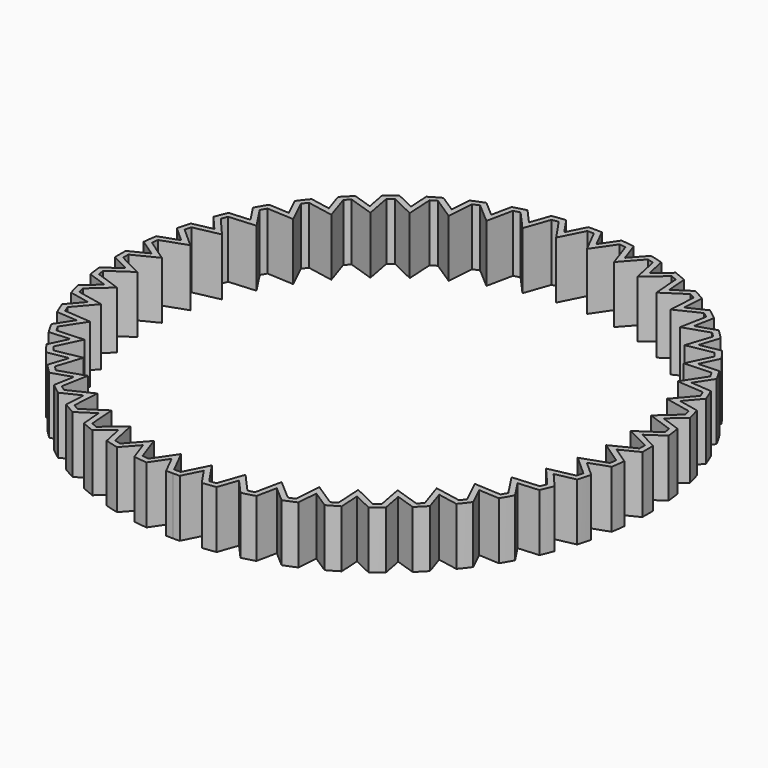
from build123d import *

# Parameters (mm, degrees)
F2_DEPTH = 5.1


# Not quite as in the source:
# - ends of sketch curves that miss each other by under 0.0002 mm in the source are joined


with BuildPart() as f2:
    # F1 (on Top) → F2 (new body, symmetric)
    with BuildSketch(Plane.XY):
        with BuildLine():
            Line((-46.740944, 4.935179), (-43.707361, 2.864732))
            Line((-43.707361, 2.864732), (-46.985243, 1.207778))
            Line((-46.985243, 1.207778), (-46.985243, 0))
            Line((-46.985243, 0), (-46.985243, -1.207778))
            Line((-46.985243, -1.207778), (-43.707361, -2.864732))
            Line((-43.707361, -2.864732), (-46.740944, -4.935179))
            ThreePointArc((-46.740944, -4.935179), (-46.5986899783, -6.134650804), (-46.4256600093, -7.3300710015))
            Line((-46.4256600093, -7.3300710015), (-42.959516, -8.545179))
            Line((-42.959516, -8.545179), (-45.696856, -10.994052))
            ThreePointArc((-45.696856, -10.994052), (-45.3992520814, -12.1646931171), (-45.0716642771, -13.3273000819))
            Line((-45.0716642771, -13.3273000819), (-41.476621, -14.079416))
            Line((-41.476621, -14.079416), (-43.870901, -16.864633))
            ThreePointArc((-43.870901, -16.864633), (-43.4230440531, -17.9864141326), (-42.9465081363, -19.0963160606))
            Line((-42.9465081363, -19.0963160606), (-39.284051, -19.37275))
            Line((-39.284051, -19.37275), (-41.294303, -22.446655))
            ThreePointArc((-41.294303, -22.446655), (-40.7038559026, -23.5003821851), (-40.0865255496, -24.5385883364))
            Line((-40.0865255496, -24.5385883364), (-36.419319, -24.334611))
            Line((-36.419319, -24.334611), (-38.011148, -27.644609))
            ThreePointArc((-38.011148, -27.644609), (-37.2882132363, -28.6122526522), (-36.5406510894, -29.5609990723))
            Line((-36.5406510894, -29.5609990723), (-32.931442, -28.8801))
            Line((-32.931442, -28.8801), (-34.077612, -32.369556))
            ThreePointArc((-34.077612, -32.369556), (-33.2345591831, -33.2345591831), (-32.3695563878, -34.0776124082))
            Line((-32.3695563878, -34.0776124082), (-28.8801, -32.931442))
            Line((-28.8801, -32.931442), (-29.5609988987, -36.540650463))
            ThreePointArc((-29.5609988987, -36.540650463), (-28.6122526522, -37.2882132363), (-27.6446094326, -38.0111485949))
            Line((-27.6446094326, -38.0111485949), (-24.334611, -36.419319))
            Line((-24.334611, -36.419319), (-24.5385880151, -40.086525271))
            ThreePointArc((-24.5385880151, -40.086525271), (-23.5003821851, -40.7038559026), (-22.4466553416, -41.2943036285))
            Line((-22.4466553416, -41.2943036285), (-19.37275, -39.284051))
            Line((-19.37275, -39.284051), (-19.0963160124, -42.9465078358))
            ThreePointArc((-19.0963160124, -42.9465078358), (-17.9864141326, -43.4230440531), (-16.864633181, -43.8709014708))
            Line((-16.864633181, -43.8709014708), (-14.079416, -41.476621))
            Line((-14.079416, -41.476621), (-13.3272999873, -45.0716640609))
            ThreePointArc((-13.3272999873, -45.0716640609), (-12.1646931171, -45.3992520814), (-10.9940520511, -45.6968562123))
            Line((-10.9940520511, -45.6968562123), (-8.545179, -42.959516))
            Line((-8.545179, -42.959516), (-7.3302500727, -46.4256317925))
            ThreePointArc((-7.3302500727, -46.4256317925), (-6.1348308361, -46.598666277), (-4.93536, -46.740925))
            Line((-4.93536, -46.740925), (-2.864732, -43.707361))
            Line((-2.864732, -43.707361), (-1.2077776691, -46.9852436547))
            Line((-1.2077776691, -46.9852436547), (0, -47.0162901536))
            Line((0, -47.0162901536), (1.2077776691, -46.9852436547))
            Line((1.2077776691, -46.9852436547), (2.864732, -43.707361))
            Line((2.864732, -43.707361), (4.93536, -46.740925))
            ThreePointArc((4.93536, -46.740925), (6.1348308361, -46.598666277), (7.330249961, -46.4256317533))
            Line((7.330249961, -46.4256317533), (8.545179, -42.959516))
            Line((8.545179, -42.959516), (10.994052, -45.696856))
            ThreePointArc((10.994052, -45.696856), (12.1646931171, -45.3992520814), (13.3273000819, -45.0716642771))
            Line((13.3273000819, -45.0716642771), (14.079416, -41.476621))
            Line((14.079416, -41.476621), (16.8646331123, -43.8709010965))
            ThreePointArc((16.8646331123, -43.8709010965), (17.9864141326, -43.4230440531), (19.0963160606, -42.9465081363))
            Line((19.0963160606, -42.9465081363), (19.37275, -39.284051))
            Line((19.37275, -39.284051), (22.4466552794, -41.2943031827))
            ThreePointArc((22.4466552794, -41.2943031827), (23.5003821851, -40.7038559026), (24.5385883364, -40.0865255496))
            Line((24.5385883364, -40.0865255496), (24.334611, -36.419319))
            Line((24.334611, -36.419319), (27.644609, -38.011148))
            ThreePointArc((27.644609, -38.011148), (28.6122526522, -37.2882132363), (29.5609990723, -36.5406510894))
            Line((29.5609990723, -36.5406510894), (28.8801, -32.931442))
            Line((28.8801, -32.931442), (32.369556, -34.077612))
            ThreePointArc((32.369556, -34.077612), (33.2345591831, -33.2345591831), (34.0776124082, -32.3695563878))
            Line((34.0776124082, -32.3695563878), (32.931442, -28.8801))
            Line((32.931442, -28.8801), (36.540651, -29.560999))
            ThreePointArc((36.540651, -29.560999), (37.2882132363, -28.6122526522), (38.0111485949, -27.6446094326))
            Line((38.0111485949, -27.6446094326), (36.419319, -24.334611))
            Line((36.419319, -24.334611), (40.086525, -24.538588))
            ThreePointArc((40.086525, -24.538588), (40.7038559026, -23.5003821851), (41.2943036285, -22.4466553416))
            Line((41.2943036285, -22.4466553416), (39.284051, -19.37275))
            Line((39.284051, -19.37275), (42.946508, -19.096316))
            ThreePointArc((42.946508, -19.096316), (43.4230440531, -17.9864141326), (43.8709014708, -16.864633181))
            Line((43.8709014708, -16.864633181), (41.476621, -14.079416))
            Line((41.476621, -14.079416), (45.071664, -13.3273))
            ThreePointArc((45.071664, -13.3273), (45.3992520814, -12.1646931171), (45.6968562123, -10.9940520511))
            Line((45.6968562123, -10.9940520511), (42.959516, -8.545179))
            Line((42.959516, -8.545179), (46.42566, -7.330071))
            ThreePointArc((46.42566, -7.330071), (46.5986899783, -6.134650804), (46.7409441102, -4.9351790116))
            Line((46.7409441102, -4.9351790116), (43.707361, -2.864732))
            Line((43.707361, -2.864732), (46.985243, -1.207778))
            Line((46.985243, -1.207778), (46.985243, 0))
            Line((46.985243, 0), (46.985243, 1.207778))
            Line((46.985243, 1.207778), (43.707361, 2.864732))
            Line((43.707361, 2.864732), (46.740944, 4.935179))
            ThreePointArc((46.740944, 4.935179), (46.5986899783, 6.134650804), (46.4256600093, 7.3300710015))
            Line((46.4256600093, 7.3300710015), (42.959516, 8.545179))
            Line((42.959516, 8.545179), (45.696856, 10.994052))
            ThreePointArc((45.696856, 10.994052), (45.3992520814, 12.1646931171), (45.0716642771, 13.3273000819))
            Line((45.0716642771, 13.3273000819), (41.476621, 14.079416))
            Line((41.476621, 14.079416), (43.870901, 16.864633))
            ThreePointArc((43.870901, 16.864633), (43.4230440531, 17.9864141326), (42.9465081363, 19.0963160606))
            Line((42.9465081363, 19.0963160606), (39.284051, 19.37275))
            Line((39.284051, 19.37275), (41.294303, 22.446655))
            ThreePointArc((41.294303, 22.446655), (40.7038559026, 23.5003821851), (40.0865255496, 24.5385883364))
            Line((40.0865255496, 24.5385883364), (36.419319, 24.334611))
            Line((36.419319, 24.334611), (38.011148, 27.644609))
            ThreePointArc((38.011148, 27.644609), (37.2882132363, 28.6122526522), (36.5406510894, 29.5609990723))
            Line((36.5406510894, 29.5609990723), (32.931442, 28.8801))
            Line((32.931442, 28.8801), (34.077612, 32.369556))
            ThreePointArc((34.077612, 32.369556), (33.2345591831, 33.2345591831), (32.3695563878, 34.0776124082))
            Line((32.3695563878, 34.0776124082), (28.8801, 32.931442))
            Line((28.8801, 32.931442), (29.5609988987, 36.540650463))
            ThreePointArc((29.5609988987, 36.540650463), (28.6122526522, 37.2882132363), (27.6446094326, 38.0111485949))
            Line((27.6446094326, 38.0111485949), (24.334611, 36.419319))
            Line((24.334611, 36.419319), (24.5385880151, 40.086525271))
            ThreePointArc((24.5385880151, 40.086525271), (23.5003821851, 40.7038559026), (22.4466553416, 41.2943036285))
            Line((22.4466553416, 41.2943036285), (19.37275, 39.284051))
            Line((19.37275, 39.284051), (19.0963160124, 42.9465078358))
            ThreePointArc((19.0963160124, 42.9465078358), (17.9864141326, 43.4230440531), (16.864633181, 43.8709014708))
            Line((16.864633181, 43.8709014708), (14.079416, 41.476621))
            Line((14.079416, 41.476621), (13.3272999873, 45.0716640609))
            ThreePointArc((13.3272999873, 45.0716640609), (12.1646931171, 45.3992520814), (10.9940520511, 45.6968562123))
            Line((10.9940520511, 45.6968562123), (8.545179, 42.959516))
            Line((8.545179, 42.959516), (7.3302500727, 46.4256317925))
            ThreePointArc((7.3302500727, 46.4256317925), (6.1348308361, 46.598666277), (4.93536, 46.740925))
            Line((4.93536, 46.740925), (2.864732, 43.707361))
            Line((2.864732, 43.707361), (1.2077776691, 46.9852436547))
            Line((1.2077776691, 46.9852436547), (0, 47.0162901536))
            Line((0, 47.0162901536), (-1.2077776691, 46.9852436547))
            Line((-1.2077776691, 46.9852436547), (-2.8647316691, 43.7073616547))
            Line((-2.8647316691, 43.7073616547), (-4.93536, 46.740925))
            ThreePointArc((-4.93536, 46.740925), (-6.1348308361, 46.598666277), (-7.330249961, 46.4256317533))
            Line((-7.330249961, 46.4256317533), (-8.545179, 42.959516))
            Line((-8.545179, 42.959516), (-10.994052, 45.696856))
            ThreePointArc((-10.994052, 45.696856), (-12.1646930606, 45.3992518705), (-13.32730002, 45.0716640678))
            Line((-13.32730002, 45.0716640678), (-14.079416, 41.476621))
            Line((-14.079416, 41.476621), (-16.864633, 43.870901))
            ThreePointArc((-16.864633, 43.870901), (-17.9864140039, 43.4230437425), (-19.096315924, 42.9465078291))
            Line((-19.096315924, 42.9465078291), (-19.37275, 39.284051))
            Line((-19.37275, 39.284051), (-22.446655, 41.294303))
            ThreePointArc((-22.446655, 41.294303), (-23.500382017, 40.7038556115), (-24.5385881609, 40.0865252629))
            Line((-24.5385881609, 40.0865252629), (-24.334611, 36.419319))
            Line((-24.334611, 36.419319), (-27.644609, 38.011148))
            ThreePointArc((-27.644609, 38.011148), (-28.6122522044, 37.2882126527), (-29.5609986097, 36.5406505175))
            Line((-29.5609986097, 36.5406505175), (-28.8801, 32.931442))
            Line((-28.8801, 32.931442), (-32.369556, 34.077612))
            ThreePointArc((-32.369556, 34.077612), (-33.2345589453, 33.2345589453), (-34.0776121645, 32.3695561562))
            Line((-34.0776121645, 32.3695561562), (-32.931442, 28.8801))
            Line((-32.931442, 28.8801), (-36.540651, 29.560999))
            ThreePointArc((-36.540651, 29.560999), (-37.2882131451, 28.6122525822), (-38.0111485019, 27.644609365))
            Line((-38.0111485019, 27.644609365), (-36.419319, 24.334611))
            Line((-36.419319, 24.334611), (-40.086525, 24.538588))
            ThreePointArc((-40.086525, 24.538588), (-40.7038556115, 23.500382017), (-41.2943033331, 22.4466551811))
            Line((-41.2943033331, 22.4466551811), (-39.284051, 19.37275))
            Line((-39.284051, 19.37275), (-42.946508, 19.096316))
            ThreePointArc((-42.946508, 19.096316), (-43.4230439153, 17.9864140755), (-43.8709013315, 16.8646331275))
            Line((-43.8709013315, 16.8646331275), (-41.476621, 14.079416))
            Line((-41.476621, 14.079416), (-45.071664, 13.3273))
            ThreePointArc((-45.071664, 13.3273), (-45.3992517567, 12.1646930301), (-45.6968558854, 10.9940519724))
            Line((-45.6968558854, 10.9940519724), (-42.959516, 8.545179))
            Line((-42.959516, 8.545179), (-46.42566, 7.330071))
            ThreePointArc((-46.42566, 7.330071), (-46.598689645, 6.1346507601), (-46.740944, 4.935179))
        make_face()
        with BuildLine():
            Line((-5.4220195115, 45.6801049272), (-2.7361214918, 41.7451424229))
            Line((-2.7361214918, 41.7451424229), (-0.5869250263, 45.9968068679))
            Line((-0.5869250263, 45.9968068679), (0, 45.9968068679))
            Line((0, 45.9968068679), (0.5869250263, 45.9968068679))
            Line((0.5869250263, 45.9968068679), (2.7361214918, 41.7451424229))
            Line((2.7361214918, 41.7451424229), (5.4220195115, 45.6801049272))
            ThreePointArc((5.4220195115, 45.6801049272), (6.0043046559, 45.607221), (6.5856126633, 45.52691498))
            Line((6.5856126633, 45.52691498), (8.1615477089, 41.0308714443))
            Line((8.1615477089, 41.0308714443), (11.3380832459, 44.5815895855))
            ThreePointArc((11.3380832459, 44.5815895855), (11.9058739168, 44.4333258717), (12.4717269771, 44.2778308858))
            Line((12.4717269771, 44.2778308858), (13.4473280598, 39.6145499373))
            Line((13.4473280598, 39.6145499373), (17.0601497389, 42.7202708524))
            ThreePointArc((17.0601497389, 42.7202708524), (17.6037306142, 42.4991641119), (18.1444465413, 42.2711407636))
            Line((18.1444465413, 42.2711407636), (18.5030205002, 37.5204144542))
            Line((18.5030205002, 37.5204144542), (22.4903118144, 40.1279967767))
            ThreePointArc((22.4903118144, 40.1279967767), (23.0003819809, 39.8378301427), (23.506708912, 39.5411800263))
            Line((23.506708912, 39.5411800263), (23.2421216274, 34.7842931877))
            Line((23.2421216274, 34.7842931877), (27.5356584306, 36.849121141))
            ThreePointArc((27.5356584306, 36.849121141), (28.0034910581, 36.4948595052), (28.4667659651, 36.1346581171))
            Line((28.4667659651, 36.1346581171), (27.5835430367, 31.4530021111))
            Line((27.5835430367, 31.4530021111), (32.109862911, 32.9397473374))
            ThreePointArc((32.109862911, 32.9397473374), (32.5274521116, 32.5274521116), (32.9397475781, 32.1098631457))
            Line((32.9397475781, 32.1098631457), (31.4530021111, 27.5835430367))
            Line((31.4530021111, 27.5835430367), (36.1346582271, 28.4667656396))
            ThreePointArc((36.1346582271, 28.4667656396), (36.4948595052, 28.0034910581), (36.8491215365, 27.5356591302))
            Line((36.8491215365, 27.5356591302), (34.7842931877, 23.2421216274))
            Line((34.7842931877, 23.2421216274), (39.5411797373, 23.5067087403))
            ThreePointArc((39.5411797373, 23.5067087403), (39.8378301427, 23.0003819809), (40.1279970699, 22.4903119788))
            Line((40.1279970699, 22.4903119788), (37.5204144542, 18.5030205002))
            Line((37.5204144542, 18.5030205002), (42.271140665, 18.1444463929))
            ThreePointArc((42.271140665, 18.1444463929), (42.4991641119, 17.6037306142), (42.7202711284, 17.0601499542))
            Line((42.7202711284, 17.0601499542), (39.6145499373, 13.4473280598))
            Line((39.6145499373, 13.4473280598), (44.2778305456, 12.4717269452))
            ThreePointArc((44.2778305456, 12.4717269452), (44.4333258717, 11.9058739168), (44.5815898122, 11.3380832401))
            Line((44.5815898122, 11.3380832401), (41.0309340793, 8.1616037433))
            Line((41.0309340793, 8.1616037433), (45.5269361782, 6.585463768))
            ThreePointArc((45.5269361782, 6.585463768), (45.6072406867, 6.0041551186), (45.6801227556, 5.4218693069))
            Line((45.6801227556, 5.4218693069), (41.7450671545, 2.7361595396))
            Line((41.7450671545, 2.7361595396), (45.9969190154, 0.5868683362))
            Line((45.9969190154, 0.5868683362), (45.9969190154, 0))
            Line((45.9969190154, 0), (45.9969190154, -0.5868683362))
            Line((45.9969190154, -0.5868683362), (41.7450671545, -2.7361595396))
            Line((41.7450671545, -2.7361595396), (45.6801224217, -5.4218692673))
            ThreePointArc((45.6801224217, -5.4218692673), (45.6072406867, -6.0041551186), (45.526936511, -6.5854638161))
            Line((45.526936511, -6.5854638161), (41.0309340793, -8.1616037433))
            Line((41.0309340793, -8.1616037433), (44.5815894864, -11.3380831572))
            ThreePointArc((44.5815894864, -11.3380831572), (44.4333258717, -11.9058739168), (44.2778308692, -12.4717270363))
            Line((44.2778308692, -12.4717270363), (39.6145499373, -13.4473280598))
            Line((39.6145499373, -13.4473280598), (42.7202709899, -17.0601498989))
            ThreePointArc((42.7202709899, -17.0601498989), (42.4991641119, -17.6037306142), (42.2711408021, -18.1444464517))
            Line((42.2711408021, -18.1444464517), (37.5204144542, -18.5030205002))
            Line((37.5204144542, -18.5030205002), (40.1279967767, -22.4903118144))
            ThreePointArc((40.1279967767, -22.4903118144), (39.8378301427, -23.0003819809), (39.5411800263, -23.506708912))
            Line((39.5411800263, -23.506708912), (34.7842931877, -23.2421216274))
            Line((34.7842931877, -23.2421216274), (36.8491214444, -27.5356590614))
            ThreePointArc((36.8491214444, -27.5356590614), (36.4948595052, -28.0034910581), (36.1346583174, -28.4667657108))
            Line((36.1346583174, -28.4667657108), (31.4530021111, -27.5835430367))
            Line((31.4530021111, -27.5835430367), (32.9397473374, -32.109862911))
            ThreePointArc((32.9397473374, -32.109862911), (32.5274521116, -32.5274521116), (32.1098631457, -32.9397475781))
            Line((32.1098631457, -32.9397475781), (27.5835430367, -31.4530021111))
            Line((27.5835430367, -31.4530021111), (28.4667655099, -36.1346575392))
            ThreePointArc((28.4667655099, -36.1346575392), (28.0034910581, -36.4948595052), (27.5356588709, -36.8491217303))
            Line((27.5356588709, -36.8491217303), (23.2421216274, -34.7842931877))
            Line((23.2421216274, -34.7842931877), (23.5067087403, -39.5411797373))
            ThreePointArc((23.5067087403, -39.5411797373), (23.0003819809, -39.8378301427), (22.4903119788, -40.1279970699))
            Line((22.4903119788, -40.1279970699), (18.5030205002, -37.5204144542))
            Line((18.5030205002, -37.5204144542), (18.1444464087, -42.2711404547))
            ThreePointArc((18.1444464087, -42.2711404547), (17.6037306142, -42.4991641119), (17.0601498636, -42.7202711646))
            Line((17.0601498636, -42.7202711646), (13.4473280598, -39.6145499373))
            Line((13.4473280598, -39.6145499373), (12.471726918, -44.2778306757))
            ThreePointArc((12.471726918, -44.2778306757), (11.9058739168, -44.4333258717), (11.3380832997, -44.5815897971))
            Line((11.3380832997, -44.5815897971), (8.1615477089, -41.0308714443))
            Line((8.1615477089, -41.0308714443), (6.5856126633, -45.52691498))
            ThreePointArc((6.5856126633, -45.52691498), (6.0043046559, -45.607221), (5.4220195115, -45.6801049272))
            Line((5.4220195115, -45.6801049272), (2.7361214918, -41.7451424229))
            Line((2.7361214918, -41.7451424229), (0.5869250263, -45.9968068679))
            Line((0.5869250263, -45.9968068679), (0, -45.9968068679))
            Line((0, -45.9968068679), (-0.5869250263, -45.9968068679))
            Line((-0.5869250263, -45.9968068679), (-2.7361214918, -41.7451424229))
            Line((-2.7361214918, -41.7451424229), (-5.4220195115, -45.6801049272))
            ThreePointArc((-5.4220195115, -45.6801049272), (-6.0043046559, -45.607221), (-6.5856126633, -45.52691498))
            Line((-6.5856126633, -45.52691498), (-8.1615477089, -41.0308714443))
            Line((-8.1615477089, -41.0308714443), (-11.3380832459, -44.5815895855))
            ThreePointArc((-11.3380832459, -44.5815895855), (-11.9058739168, -44.4333258717), (-12.4717269771, -44.2778308858))
            Line((-12.4717269771, -44.2778308858), (-13.4473280598, -39.6145499373))
            Line((-13.4473280598, -39.6145499373), (-17.0601497389, -42.7202708524))
            ThreePointArc((-17.0601497389, -42.7202708524), (-17.6037306142, -42.4991641119), (-18.1444465413, -42.2711407636))
            Line((-18.1444465413, -42.2711407636), (-18.5030205002, -37.5204144542))
            Line((-18.5030205002, -37.5204144542), (-22.4903118144, -40.1279967767))
            ThreePointArc((-22.4903118144, -40.1279967767), (-23.0003819809, -39.8378301427), (-23.506708912, -39.5411800263))
            Line((-23.506708912, -39.5411800263), (-23.2421216274, -34.7842931877))
            Line((-23.2421216274, -34.7842931877), (-27.5356584306, -36.849121141))
            ThreePointArc((-27.5356584306, -36.849121141), (-28.0034910581, -36.4948595052), (-28.4667659651, -36.1346581171))
            Line((-28.4667659651, -36.1346581171), (-27.5835430367, -31.4530021111))
            Line((-27.5835430367, -31.4530021111), (-32.109862911, -32.9397473374))
            ThreePointArc((-32.109862911, -32.9397473374), (-32.5274521116, -32.5274521116), (-32.9397475781, -32.1098631457))
            Line((-32.9397475781, -32.1098631457), (-31.4530021111, -27.5835430367))
            Line((-31.4530021111, -27.5835430367), (-36.1346582271, -28.4667656396))
            ThreePointArc((-36.1346582271, -28.4667656396), (-36.4948595052, -28.0034910581), (-36.8491215365, -27.5356591302))
            Line((-36.8491215365, -27.5356591302), (-34.7842931877, -23.2421216274))
            Line((-34.7842931877, -23.2421216274), (-39.5411797373, -23.5067087403))
            ThreePointArc((-39.5411797373, -23.5067087403), (-39.8378301427, -23.0003819809), (-40.1279970699, -22.4903119788))
            Line((-40.1279970699, -22.4903119788), (-37.5204144542, -18.5030205002))
            Line((-37.5204144542, -18.5030205002), (-42.271140665, -18.1444463929))
            ThreePointArc((-42.271140665, -18.1444463929), (-42.4991641119, -17.6037306142), (-42.7202711284, -17.0601499542))
            Line((-42.7202711284, -17.0601499542), (-39.6145499373, -13.4473280598))
            Line((-39.6145499373, -13.4473280598), (-44.2778305456, -12.4717269452))
            ThreePointArc((-44.2778305456, -12.4717269452), (-44.4333258717, -11.9058739168), (-44.5815898122, -11.3380832401))
            Line((-44.5815898122, -11.3380832401), (-41.0309340793, -8.1616037433))
            Line((-41.0309340793, -8.1616037433), (-45.5269361782, -6.585463768))
            ThreePointArc((-45.5269361782, -6.585463768), (-45.6072406867, -6.0041551186), (-45.6801227556, -5.4218693069))
            Line((-45.6801227556, -5.4218693069), (-41.7450671545, -2.7361595396))
            Line((-41.7450671545, -2.7361595396), (-45.9969190154, -0.5868683362))
            Line((-45.9969190154, -0.5868683362), (-45.9969190154, 0))
            Line((-45.9969190154, 0), (-45.9969190154, 0.5868683362))
            Line((-45.9969190154, 0.5868683362), (-41.7450671545, 2.7361595396))
            Line((-41.7450671545, 2.7361595396), (-45.6801224217, 5.4218692673))
            ThreePointArc((-45.6801224217, 5.4218692673), (-45.6072403534, 6.0041550747), (-45.5269361782, 6.585463768))
            Line((-45.5269361782, 6.585463768), (-41.0309340793, 8.1616037433))
            Line((-41.0309340793, 8.1616037433), (-44.5815894864, 11.3380831572))
            ThreePointArc((-44.5815894864, 11.3380831572), (-44.433325547, 11.9058738298), (-44.2778305456, 12.4717269452))
            Line((-44.2778305456, 12.4717269452), (-39.6145499373, 13.4473280598))
            Line((-39.6145499373, 13.4473280598), (-42.7202709899, 17.0601498989))
            ThreePointArc((-42.7202709899, 17.0601498989), (-42.4991639741, 17.6037305572), (-42.271140665, 18.1444463929))
            Line((-42.271140665, 18.1444463929), (-37.5204144542, 18.5030205002))
            Line((-37.5204144542, 18.5030205002), (-40.1279967767, 22.4903118144))
            ThreePointArc((-40.1279967767, 22.4903118144), (-39.8378298516, 23.0003818128), (-39.5411797373, 23.5067087403))
            Line((-39.5411797373, 23.5067087403), (-34.7842931877, 23.2421216274))
            Line((-34.7842931877, 23.2421216274), (-36.8491214444, 27.5356590614))
            ThreePointArc((-36.8491214444, 27.5356590614), (-36.494859414, 28.0034909881), (-36.1346582271, 28.4667656396))
            Line((-36.1346582271, 28.4667656396), (-31.4530021111, 27.5835430367))
            Line((-31.4530021111, 27.5835430367), (-32.9397473374, 32.109862911))
            ThreePointArc((-32.9397473374, 32.109862911), (-32.5274518739, 32.5274518739), (-32.109862911, 32.9397473374))
            Line((-32.109862911, 32.9397473374), (-27.5835430367, 31.4530021111))
            Line((-27.5835430367, 31.4530021111), (-28.4667655099, 36.1346575392))
            ThreePointArc((-28.4667655099, 36.1346575392), (-28.0034906103, 36.4948589216), (-27.5356584306, 36.849121141))
            Line((-27.5356584306, 36.849121141), (-23.2421216274, 34.7842931877))
            Line((-23.2421216274, 34.7842931877), (-23.5067087403, 39.5411797373))
            ThreePointArc((-23.5067087403, 39.5411797373), (-23.0003818128, 39.8378298516), (-22.4903118144, 40.1279967767))
            Line((-22.4903118144, 40.1279967767), (-18.5030205002, 37.5204144542))
            Line((-18.5030205002, 37.5204144542), (-18.1444464087, 42.2711404547))
            ThreePointArc((-18.1444464087, 42.2711404547), (-17.6037304856, 42.4991638013), (-17.0601497389, 42.7202708524))
            Line((-17.0601497389, 42.7202708524), (-13.4473280598, 39.6145499373))
            Line((-13.4473280598, 39.6145499373), (-12.471726918, 44.2778306757))
            ThreePointArc((-12.471726918, 44.2778306757), (-11.9058738603, 44.4333256608), (-11.3380832459, 44.5815895855))
            Line((-11.3380832459, 44.5815895855), (-8.1615477089, 41.0308714443))
            Line((-8.1615477089, 41.0308714443), (-6.5856126633, 45.52691498))
            ThreePointArc((-6.5856126633, 45.52691498), (-6.0043046559, 45.607221), (-5.4220195115, 45.6801049272))
        make_face(mode=Mode.SUBTRACT)
    extrude(amount=F2_DEPTH, both=True)


solid = f2.part
